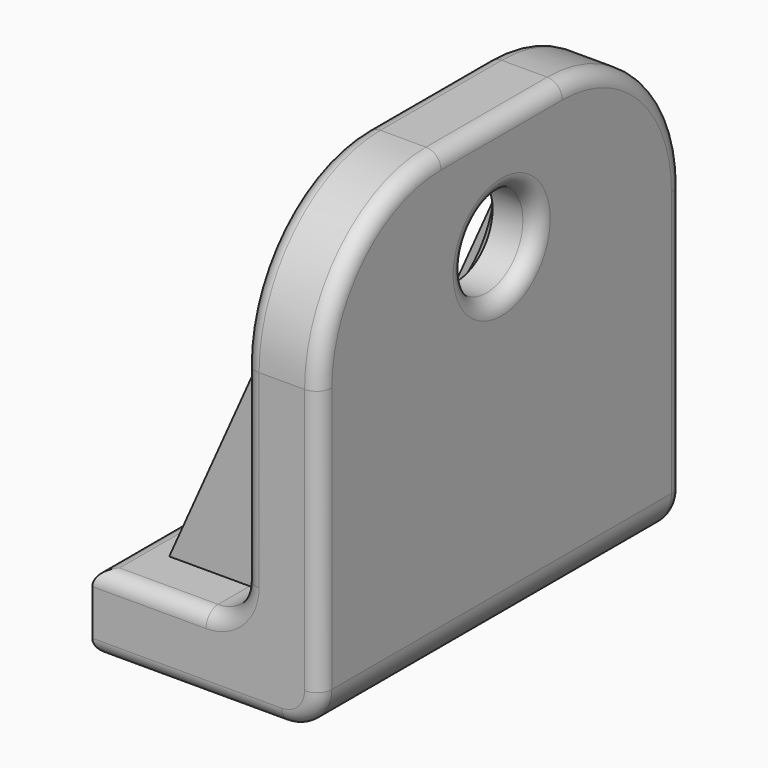
from build123d import *

# Parameters (mm, degrees)
F1_DEPTH  = 30
F2_R      = 6
F3_DEPTH  = 10
F4_R      = 10
F5_DEPTH  = 4
F7_DEPTH  = 10
F10_DEPTH = 4.8
F12_DEPTH = 2
F13_R     = 20
F14_R     = 1.99999
F14_2_R   = 1.99999


# Not quite as in the source:
# - a fillet or chamfer is up to 0.001 mm smaller than in the source, because OpenCascade refuses the exact size
# - a pattern or mirror of a feature is missing from the dataset's text; its kind, count and spacing are read off the source's solid


with BuildPart() as f1:
    # F0 (on Front) → F1 (new body, symmetric)
    with BuildSketch(Plane.XZ):
        with BuildLine():
            Line((0, 10), (0, 0))
            Line((0, 0), (25, 0))
            ThreePointArc((25, 0), (28.5355339059, 1.4644660941), (30, 5))
            Line((30, 5), (30, 60))
            Line((30, 60), (20, 60))
            Line((20, 60), (20, 15))
            ThreePointArc((20, 15), (18.5355339059, 11.4644660941), (15, 10))
            Line((15, 10), (0, 10))
        make_face()
    extrude(amount=F1_DEPTH, both=True)

    # F2 (on face) → F3 (cut, through all)
    with BuildSketch(Plane.YZ.offset(30)):
        with Locations((0, 45)):
            Circle(F2_R)
    extrude(amount=-F3_DEPTH, mode=Mode.SUBTRACT)

    # F4 (on face) → F5 (cut)
    with BuildSketch(Plane(origin=(20, 0, 0), x_dir=(0, -1, 0), z_dir=(-1, 0, 0))):
        with Locations((0, 45)):
            Circle(F4_R)
    extrude(amount=-F5_DEPTH, mode=Mode.SUBTRACT)

    # F6 (on face) → F7 (cut, through all)
    with BuildSketch(Plane.XY.offset(10)):
        with BuildLine():
            Line((0, -5), (7.5000035577, -5))
            ThreePointArc((7.5000035577, -5), (12.5000035577, 0), (7.5000035577, 5))
            Line((7.5000035577, 5), (0, 5))
            Line((0, 5), (0, -5))
        make_face()
    extrude(amount=-F7_DEPTH, mode=Mode.SUBTRACT)

    # F13
    f13_edges = [f1.edges().sort_by_distance(p)[0] for p in [
        (25, 30, 60),
        (25, -30, 60),
    ]]
    fillet(f13_edges, radius=F13_R)

    # F14 (radius 2 in the source; OpenCascade refuses exactly that, so slightly less here)
    f14_edges = [f1.edges().sort_by_distance(p)[0] for p in [
        (7.5, -30, 10),
        (0, -17.5, 10),
        (0, 17.5, 10),
        (20, 30, 27.5),
        (20, 24.142136, 54.142136),
        (20, 0, 15),
        (20, 0, 60),
        (20, -30, 27.5),
        (20, -24.142136, 54.142136),
        (20, 10, 45),
        (30, 30, 22.5),
        (30, 24.142136, 54.142136),
        (30, 0, 5),
        (30, 0, 60),
        (30, -30, 22.5),
        (30, -24.142136, 54.142136),
        (30, -6, 45),
        (0, 17.5, 0),
        (3.750002, 5, 0),
        (12.500004, 0, 0),
        (3.750002, -5, 0),
        (0, -17.5, 0),
        (12.5, -30, 0),
        (25, 0, 0),
        (12.5, 30, 0),
        (28.535534, -30, 1.464466),
        (18.535534, -30, 11.464466),
        (28.535534, 30, 1.464466),
        (18.535534, 30, 11.464466),
        (7.5, 30, 10),
    ]]
    fillet(f14_edges, radius=F14_R)


with BuildPart() as f10:
    # F9 (on offset) → F10 (new body, symmetric)
    with BuildSketch(Plane.XZ.offset(18)):
        with BuildLine():
            ThreePointArc((15, 10), (18.5355339059, 11.4644660941), (20, 15))
            Line((20, 15), (20, 45))
            Line((20, 45), (4.3933112174, 10))
            Line((4.3933112174, 10), (15, 10))
        make_face()
    extrude(amount=F10_DEPTH, both=True)


with BuildPart() as f10_copies_1:
    # F10_copies: instance of F10
    add(f10.part.mirror(Plane.ZX))


with BuildPart() as f12:
    # F11 (on face) → F12 (new body)
    with BuildSketch(Plane.XY.offset(10)):
        with BuildLine():
            ThreePointArc((7.5000035577, 5), (12.5000035577, 0), (7.5000035577, -5))
            Line((7.5000035577, -5), (0, -5))
            Line((0, -5), (0, -7))
            Line((0, -7), (7.5000035577, -7))
            ThreePointArc((7.5000035577, -7), (14.5000035577, 0), (7.5000035577, 7))
            Line((7.5000035577, 7), (0, 7))
            Line((0, 7), (0, 5))
            Line((0, 5), (7.5000035577, 5))
        make_face()
    extrude(amount=F12_DEPTH)

    # F14#2 (radius 2 in the source; OpenCascade refuses exactly that, so slightly less here)
    f14_2_edges = [f12.edges().sort_by_distance(p)[0] for p in [
        (3.750002, -7, 12),
        (14.500004, 0, 12),
        (3.750002, 7, 12),
    ]]
    fillet(f14_2_edges, radius=F14_2_R)


solid = Compound([f1.part, f10.part, f10_copies_1.part, f12.part])
